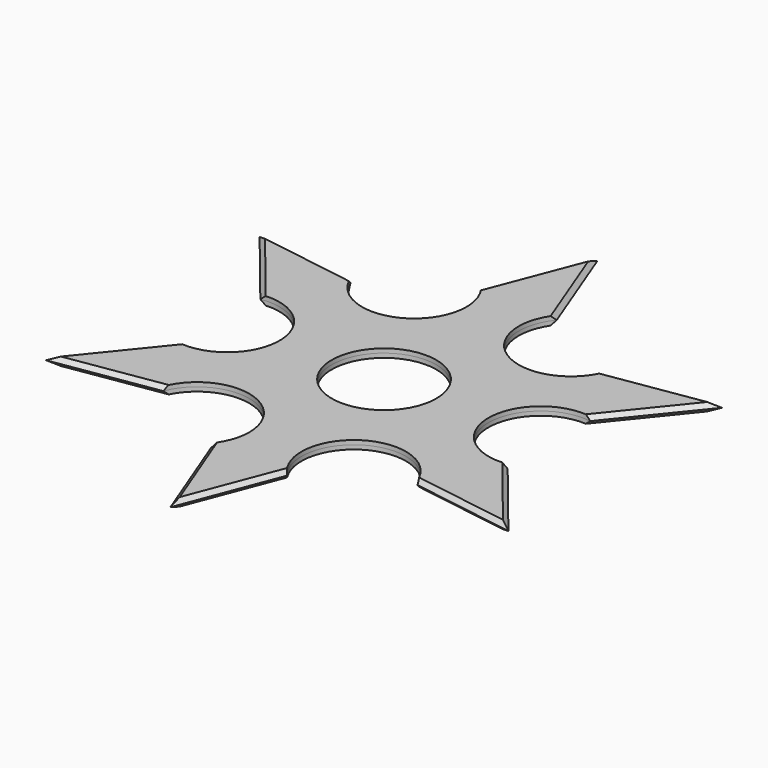
from build123d import *

# Parameters (mm, degrees)
F0_R         = 12.5
F1_DEPTH     = 1
F2_T1_DEPTH  = 53.573606434
F2_T3_DEPTH  = 53.573606434
F2_T5_DEPTH  = 53.5736064345
F2_T7_DEPTH  = 53.5736064338
F2_T9_DEPTH  = 53.573606434
F2_T11_DEPTH = 59.849360607
F2_T13_DEPTH = 53.5916397473
F2_T15_DEPTH = 53.5736064341
F2_T17_DEPTH = 53.573606434
F2_T19_DEPTH = 53.573606434
F2_T21_DEPTH = 59.8387499617
F3_DEPTH     = 1
F4_T1_DEPTH  = 40.7151914942
F4_T3_DEPTH  = 19.123558468
F4_T5_DEPTH  = 40.7151914942
F4_T7_DEPTH  = 19.1235584677
F4_T9_DEPTH  = 59.8387499623
F4_T11_DEPTH = 59.8387499618
F4_T13_DEPTH = 59.8387499617
F4_T15_DEPTH = 59.8387499618
F4_T17_DEPTH = 40.7151914942
F4_T19_DEPTH = 19.1235584677
F4_T21_DEPTH = 40.7151914943
F4_T23_DEPTH = 19.1235584676
F4_T25_DEPTH = 59.828531224
F4_T27_DEPTH = 59.849360607
F5_T1_DEPTH  = 59.8387499611
F5_T3_DEPTH  = 59.838749962
F6_T1_DEPTH  = 52.3772114997


# Not quite as in the source:
# - a fillet or chamfer that OpenCascade refuses, or shapes differently, is made with other operations: its cross-section is extruded or revolved along the edge and cut away or added
# - a feature names something its author has since deleted; it is built from what else it names


with BuildPart() as f1:
    # F0 (on Top) → F1 (new body)
    with BuildSketch(Plane.XY):
        with BuildLine():
            ThreePointArc((12.1993091148, -43.1220058508), (12.5252728209, -21.6360831063), (31.2465952446, -32.1842211044))
            Line((31.2465952446, -32.1842211044), (37.4352447857, -33.1602540379))
            Line((37.4352447857, -33.1602540379), (64.9519052827, -37.5000000012))
            Line((64.9519052827, -37.5000000012), (47.4352447858, -15.8397459622))
            Line((47.4352447858, -15.8397459622), (47.4101819713, -15.8831560303))
            ThreePointArc((47.4101819713, -15.8831560303), (47.4189900332, -15.8568402989), (47.4277834882, -15.830519683))
            Line((47.4277834882, -15.830519683), (43.4956507006, -10.968234711))
            ThreePointArc((43.4956507006, -10.968234711), (25, -3e-10), (43.4956507, 10.9682347114))
            Line((43.4956507, 10.9682347114), (47.4277834882, 15.8305196828))
            ThreePointArc((47.4277834882, 15.8305196828), (47.4189900332, 15.8568402987), (47.4101819713, 15.8831560301))
            Line((47.4101819713, 15.8831560301), (47.4352447858, 15.8397459621))
            Line((47.4352447858, 15.8397459621), (64.9519052853, 37.4999999987))
            Line((64.9519052853, 37.4999999987), (37.4352447862, 33.1602540379))
            Line((37.4352447862, 33.1602540379), (37.4603076002, 33.1168439697))
            ThreePointArc((37.4603076002, 33.1168439697), (37.4419215393, 33.1376298408), (37.4235239447, 33.1584055041))
            Line((37.4235239447, 33.1584055041), (31.2465952455, 32.1842211051))
            ThreePointArc((31.2465952455, 32.1842211051), (12.500000001, 21.6506350947), (12.2490554557, 43.152455816))
            Line((12.2490554557, 43.152455816), (10.0042595438, 48.988925187))
            ThreePointArc((10.0042595437, 48.988925187), (9.9770684942, 48.9944701396), (9.9498743714, 49))
            Line((9.9498743714, 49), (10.0000000003, 49))
            Line((10.0000000003, 49), (3e-10, 75))
            Line((3e-10, 75), (-9.9999999997, 49))
            Line((-9.9999999997, 49), (-9.9498743707, 49))
            ThreePointArc((-9.9498743707, 49), (-9.9770684936, 48.9944701396), (-10.0042595431, 48.988925187))
            Line((-10.0042595431, 48.988925187), (-12.2490554551, 43.1524558158))
            ThreePointArc((-12.2490554551, 43.1524558158), (-12.4999999997, 21.6506350948), (-31.2465952441, 32.1842211045))
            Line((-31.2465952441, 32.1842211045), (-37.4352447851, 33.1602540377))
            Line((-37.4352447851, 33.1602540377), (-64.951905283, 37.5000000002))
            Line((-64.951905283, 37.5000000002), (-47.4352447851, 15.839745962))
            Line((-47.4352447851, 15.839745962), (-47.4101819706, 15.8831560301))
            ThreePointArc((-47.4101819706, 15.8831560301), (-47.4189900325, 15.8568402987), (-47.4277834875, 15.8305196828))
            Line((-47.4277834875, 15.8305196828), (-43.4956506999, 10.9682347111))
            ThreePointArc((-43.4956506999, 10.9682347111), (-24.9999999998, 0), (-43.4956506997, -10.9682347113))
            Line((-43.4956506997, -10.9682347113), (-47.4277834875, -15.830519683))
            ThreePointArc((-47.4277834875, -15.830519683), (-47.4189900326, -15.8568402989), (-47.4101819706, -15.8831560303))
            Line((-47.4101819706, -15.8831560303), (-47.4352447851, -15.8397459622))
            Line((-47.4352447851, -15.8397459622), (-64.9519052836, -37.5))
            Line((-64.9519052836, -37.5), (-37.4352447851, -33.1602540379))
            Line((-37.4352447851, -33.1602540379), (-37.4603075996, -33.1168439699))
            ThreePointArc((-37.4603075996, -33.1168439699), (-37.4419215386, -33.1376298409), (-37.4235239441, -33.1584055043))
            Line((-37.4235239441, -33.1584055043), (-31.2465952444, -32.1842211048))
            ThreePointArc((-31.2465952444, -32.1842211048), (-12.4748304406, -21.6652058125), (-12.2988061822, -43.1825906916))
            Line((-12.2988061822, -43.1825906916), (-10.058717508, -48.977772531))
            ThreePointArc((-10.058717508, -48.977772531), (-10.0043021126, -48.9889164938), (-9.9498743711, -49))
            Line((-9.9498743711, -49), (-10.0501256289, -49))
            Line((-10.0501256289, -49), (0, -75))
            Line((0, -75), (9.9498743711, -49))
            Line((9.9498743711, -49), (12.1993091148, -43.1220058508))
        make_face()
        Circle(F0_R, mode=Mode.SUBTRACT)
    extrude(amount=F1_DEPTH)

    # F2: chamfer of 5 on 11 edges, made by hand

    # F2_s2 → F2_t1 (cut)
    with BuildSketch(Plane(origin=(-10.5129640229, 27.3337064595, 0), x_dir=(0, 0, 1), z_dir=(-0.3589790793, 0.9333456062, 0))):
        Polygon((1, 21.9234309485), (-4, 26.9234309485), (1, 26.9234309485), align=None)
    extrude(amount=F2_T1_DEPTH, mode=Mode.SUBTRACT)

    # F2_s4 → F2_t3 (cut)
    with BuildSketch(Plane(origin=(29.7447679359, 77.3363966333, 0), x_dir=(0, 0, 1), z_dir=(-0.3589790793, -0.9333456062, 0))):
        Polygon((1, 21.9234309479), (-4, 26.9234309479), (1, 26.9234309479), align=None)
    extrude(amount=F2_T3_DEPTH, mode=Mode.SUBTRACT)

    # F2_s6 → F2_t5 (cut)
    with BuildSketch(Plane(origin=(81.84766809, 12.9084736504, 0), x_dir=(0, 0, 1), z_dir=(-0.9877905451, -0.1557878009, 0))):
        Polygon((1, 21.9234309501), (-4, 26.9234309501), (1, 26.9234309501), align=None)
    extrude(amount=F2_T5_DEPTH, mode=Mode.SUBTRACT)

    # F2_s8 → F2_t7 (cut)
    with BuildSketch(Plane(origin=(18.4152021646, 22.771347143, 0), x_dir=(0, 0, 1), z_dir=(0.6288114659, 0.7775578052, 0))):
        Polygon((1, 21.9234309459), (-4, 26.9234309459), (1, 26.9234309459), align=None)
    extrude(amount=F2_T7_DEPTH, mode=Mode.SUBTRACT)

    # F2_s10 → F2_t9 (cut)
    with BuildSketch(Plane(origin=(52.1029001483, -64.427922981, 0), x_dir=(0, 0, 1), z_dir=(-0.6288114658, 0.7775578053, 0))):
        Polygon((1, 21.9234309512), (-4, 26.9234309512), (1, 26.9234309512), align=None)
    extrude(amount=F2_T9_DEPTH, mode=Mode.SUBTRACT)

    # F2_s12 → F2_t11 (cut)
    with BuildSketch(Plane(origin=(-8.2401320813, -21.5322752955, 0), x_dir=(0, 0, 1), z_dir=(-0.3574100383, -0.9339475705, 0))):
        Polygon((1, -21.8057528732), (-4, -26.8057528732), (1, -26.8057528732), align=None)
    extrude(amount=F2_T11_DEPTH, mode=Mode.SUBTRACT)

    # F2_s14 → F2_t13 (cut)
    with BuildSketch(Plane(origin=(10.5359959788, -27.256962307, 0), x_dir=(0, 0, 1), z_dir=(0.3605450827, -0.9327417881, 0))):
        Polygon((1, 22.0408812024), (-4, 27.0408812024), (1, 27.0408812024), align=None)
    extrude(amount=F2_T13_DEPTH, mode=Mode.SUBTRACT)

    # F2_s16 → F2_t15 (cut)
    with BuildSketch(Plane(origin=(-81.8476680892, -12.9084736542, 0), x_dir=(0, 0, 1), z_dir=(0.9877905451, 0.155787801, 0))):
        Polygon((1, 21.9234309484), (-4, 26.9234309484), (1, 26.9234309484), align=None)
    extrude(amount=F2_T15_DEPTH, mode=Mode.SUBTRACT)

    # F2_s18 → F2_t17 (cut)
    with BuildSketch(Plane(origin=(-18.4152021622, -22.7713471426, 0), x_dir=(0, 0, 1), z_dir=(-0.6288114658, -0.7775578052, 0))):
        Polygon((1, 21.9234309477), (-4, 26.9234309477), (1, 26.9234309477), align=None)
    extrude(amount=F2_T17_DEPTH, mode=Mode.SUBTRACT)

    # F2_s20 → F2_t19 (cut)
    with BuildSketch(Plane(origin=(-52.1029001516, 64.4279229792, 0), x_dir=(0, 0, 1), z_dir=(0.6288114658, -0.7775578052, 0))):
        Polygon((1, 21.9234309489), (-4, 26.9234309489), (1, 26.9234309489), align=None)
    extrude(amount=F2_T19_DEPTH, mode=Mode.SUBTRACT)

    # F2_s22 → F2_t21 (cut)
    with BuildSketch(Plane(origin=(-81.8476680889, 12.9084736558, 0), x_dir=(0, 0, 1), z_dir=(0.9877905451, -0.155787801, 0))):
        Polygon((1, -21.9234309474), (-4, -26.9234309474), (1, -26.9234309474), align=None)
    extrude(amount=F2_T21_DEPTH, mode=Mode.SUBTRACT)

    # F6: chamfer of 5 on 1 edges, made by hand

    # F6_s2 → F6_t1 (cut)
    with BuildSketch(Plane(origin=(74.477230945, -11.7460569893, 0), x_dir=(0, 0, 1), z_dir=(-0.9877905451, 0.155787801, 0))):
        Polygon((1, -21.9234309461), (-4, -26.9234309461), (1, -26.9234309461), align=None)
    extrude(amount=F6_T1_DEPTH, mode=Mode.SUBTRACT)


with BuildPart() as f3:
    # F0 (on Top) → F3 (new body)
    with BuildSketch(Plane.XY):
        with BuildLine():
            ThreePointArc((12.1993091148, -43.1220058508), (12.5252728209, -21.6360831063), (31.2465952446, -32.1842211044))
            Line((31.2465952446, -32.1842211044), (37.4352447857, -33.1602540379))
            Line((37.4352447857, -33.1602540379), (64.9519052827, -37.5000000012))
            Line((64.9519052827, -37.5000000012), (47.4352447858, -15.8397459622))
            Line((47.4352447858, -15.8397459622), (47.4101819713, -15.8831560303))
            ThreePointArc((47.4101819713, -15.8831560303), (47.4189900332, -15.8568402989), (47.4277834882, -15.830519683))
            Line((47.4277834882, -15.830519683), (43.4956507006, -10.968234711))
            ThreePointArc((43.4956507006, -10.968234711), (25, -3e-10), (43.4956507, 10.9682347114))
            Line((43.4956507, 10.9682347114), (47.4277834882, 15.8305196828))
            ThreePointArc((47.4277834882, 15.8305196828), (47.4189900332, 15.8568402987), (47.4101819713, 15.8831560301))
            Line((47.4101819713, 15.8831560301), (47.4352447858, 15.8397459621))
            Line((47.4352447858, 15.8397459621), (64.9519052853, 37.4999999987))
            Line((64.9519052853, 37.4999999987), (37.4352447862, 33.1602540379))
            Line((37.4352447862, 33.1602540379), (37.4603076002, 33.1168439697))
            ThreePointArc((37.4603076002, 33.1168439697), (37.4419215393, 33.1376298408), (37.4235239447, 33.1584055041))
            Line((37.4235239447, 33.1584055041), (31.2465952455, 32.1842211051))
            ThreePointArc((31.2465952455, 32.1842211051), (12.500000001, 21.6506350947), (12.2490554557, 43.152455816))
            Line((12.2490554557, 43.152455816), (10.0042595438, 48.988925187))
            ThreePointArc((10.0042595437, 48.988925187), (9.9770684942, 48.9944701396), (9.9498743714, 49))
            Line((9.9498743714, 49), (10.0000000003, 49))
            Line((10.0000000003, 49), (3e-10, 75))
            Line((3e-10, 75), (-9.9999999997, 49))
            Line((-9.9999999997, 49), (-9.9498743707, 49))
            ThreePointArc((-9.9498743707, 49), (-9.9770684936, 48.9944701396), (-10.0042595431, 48.988925187))
            Line((-10.0042595431, 48.988925187), (-12.2490554551, 43.1524558158))
            ThreePointArc((-12.2490554551, 43.1524558158), (-12.4999999997, 21.6506350948), (-31.2465952441, 32.1842211045))
            Line((-31.2465952441, 32.1842211045), (-37.4352447851, 33.1602540377))
            Line((-37.4352447851, 33.1602540377), (-64.951905283, 37.5000000002))
            Line((-64.951905283, 37.5000000002), (-47.4352447851, 15.839745962))
            Line((-47.4352447851, 15.839745962), (-47.4101819706, 15.8831560301))
            ThreePointArc((-47.4101819706, 15.8831560301), (-47.4189900325, 15.8568402987), (-47.4277834875, 15.8305196828))
            Line((-47.4277834875, 15.8305196828), (-43.4956506999, 10.9682347111))
            ThreePointArc((-43.4956506999, 10.9682347111), (-24.9999999998, 0), (-43.4956506997, -10.9682347113))
            Line((-43.4956506997, -10.9682347113), (-47.4277834875, -15.830519683))
            ThreePointArc((-47.4277834875, -15.830519683), (-47.4189900326, -15.8568402989), (-47.4101819706, -15.8831560303))
            Line((-47.4101819706, -15.8831560303), (-47.4352447851, -15.8397459622))
            Line((-47.4352447851, -15.8397459622), (-64.9519052836, -37.5))
            Line((-64.9519052836, -37.5), (-37.4352447851, -33.1602540379))
            Line((-37.4352447851, -33.1602540379), (-37.4603075996, -33.1168439699))
            ThreePointArc((-37.4603075996, -33.1168439699), (-37.4419215386, -33.1376298409), (-37.4235239441, -33.1584055043))
            Line((-37.4235239441, -33.1584055043), (-31.2465952444, -32.1842211048))
            ThreePointArc((-31.2465952444, -32.1842211048), (-12.4748304406, -21.6652058125), (-12.2988061822, -43.1825906916))
            Line((-12.2988061822, -43.1825906916), (-10.058717508, -48.977772531))
            ThreePointArc((-10.058717508, -48.977772531), (-10.0043021126, -48.9889164938), (-9.9498743711, -49))
            Line((-9.9498743711, -49), (-10.0501256289, -49))
            Line((-10.0501256289, -49), (0, -75))
            Line((0, -75), (9.9498743711, -49))
            Line((9.9498743711, -49), (12.1993091148, -43.1220058508))
        make_face()
        Circle(F0_R, mode=Mode.SUBTRACT)
        with BuildLine():
            Line((47.4101819713, -15.8831560303), (47.4352447858, -15.8397459622))
            Line((47.4352447858, -15.8397459622), (47.4277834882, -15.830519683))
            ThreePointArc((47.4277834882, -15.830519683), (47.4189900332, -15.8568402989), (47.4101819713, -15.8831560303))
        make_face()
        with BuildLine():
            Line((-10.058717508, -48.977772531), (-10.0501256289, -49))
            Line((-10.0501256289, -49), (-9.9498743711, -49))
            ThreePointArc((-9.9498743711, -49), (-10.0043021126, -48.9889164938), (-10.058717508, -48.977772531))
        make_face()
        with BuildLine():
            ThreePointArc((47.4101819713, 15.8831560301), (47.4189900332, 15.8568402987), (47.4277834882, 15.8305196828))
            Line((47.4277834882, 15.8305196828), (47.4352447858, 15.8397459621))
            Line((47.4352447858, 15.8397459621), (47.4101819713, 15.8831560301))
        make_face()
        with BuildLine():
            Line((-37.4352447851, -33.1602540379), (-37.4235239441, -33.1584055043))
            ThreePointArc((-37.4235239441, -33.1584055043), (-37.4419215386, -33.1376298409), (-37.4603075996, -33.1168439699))
            Line((-37.4603075996, -33.1168439699), (-37.4352447851, -33.1602540379))
        make_face()
        with BuildLine():
            Line((37.4603076002, 33.1168439697), (37.4352447862, 33.1602540379))
            Line((37.4352447862, 33.1602540379), (37.4235239447, 33.1584055041))
            ThreePointArc((37.4235239447, 33.1584055041), (37.4419215393, 33.1376298408), (37.4603076002, 33.1168439697))
        make_face()
        with BuildLine():
            Line((-47.4277834875, -15.830519683), (-47.4352447851, -15.8397459622))
            Line((-47.4352447851, -15.8397459622), (-47.4101819706, -15.8831560303))
            ThreePointArc((-47.4101819706, -15.8831560303), (-47.4189900326, -15.8568402989), (-47.4277834875, -15.830519683))
        make_face()
        with BuildLine():
            ThreePointArc((9.9498743714, 49), (9.9770684942, 48.9944701396), (10.0042595437, 48.988925187))
            Line((10.0042595438, 48.988925187), (10.0000000003, 49))
            Line((10.0000000003, 49), (9.9498743714, 49))
        make_face()
        with BuildLine():
            Line((-47.4352447851, 15.839745962), (-47.4277834875, 15.8305196828))
            ThreePointArc((-47.4277834875, 15.8305196828), (-47.4189900325, 15.8568402987), (-47.4101819706, 15.8831560301))
            Line((-47.4101819706, 15.8831560301), (-47.4352447851, 15.839745962))
        make_face()
        with BuildLine():
            Line((-9.9498743707, 49), (-9.9999999997, 49))
            Line((-9.9999999997, 49), (-10.0042595431, 48.988925187))
            ThreePointArc((-10.0042595431, 48.988925187), (-9.9770684936, 48.9944701396), (-9.9498743707, 49))
        make_face()
    extrude(amount=-F3_DEPTH)

    # F4: chamfer of 5 on 14 edges, made by hand

    # F4_s2 → F4_t1 (cut)
    with BuildSketch(Plane(origin=(29.7447679359, 77.3363966333, 0), x_dir=(0, 0, 1), z_dir=(-0.3589790793, -0.9333456062, 0))):
        Polygon((4, 26.9234309479), (-1, 21.9234309479), (-1, 26.9234309479), align=None)
    extrude(amount=F4_T1_DEPTH, mode=Mode.SUBTRACT)

    # F4_s4 → F4_t3 (cut)
    with BuildSketch(Plane(origin=(15.1288659793, 39.3350515467, 0), x_dir=(0, 0, 1), z_dir=(-0.3589790793, -0.9333456062, 0))):
        Polygon((4, 26.9234309477), (-1, 21.9234309477), (-1, 26.9234309477), align=None)
    extrude(amount=F4_T3_DEPTH, mode=Mode.SUBTRACT)

    # F4_s6 → F4_t5 (cut)
    with BuildSketch(Plane(origin=(-15.1288659793, 39.3350515463, 0), x_dir=(0, 0, 1), z_dir=(-0.3589790793, 0.9333456062, 0))):
        Polygon((4, 26.9234309485), (-1, 21.9234309485), (-1, 26.9234309485), align=None)
    extrude(amount=F4_T5_DEPTH, mode=Mode.SUBTRACT)

    # F4_s8 → F4_t7 (cut)
    with BuildSketch(Plane(origin=(-8.2639085674, 21.4861622756, 0), x_dir=(0, 0, 1), z_dir=(-0.3589790793, 0.9333456062, 0))):
        Polygon((4, 26.9234309483), (-1, 21.9234309483), (-1, 26.9234309483), align=None)
    extrude(amount=F4_T7_DEPTH, mode=Mode.SUBTRACT)

    # F4_s10 → F4_t9 (cut)
    with BuildSketch(Plane(origin=(81.84766809, 12.9084736504, 0), x_dir=(0, 0, 1), z_dir=(-0.9877905451, -0.1557878009, 0))):
        Polygon((4, 26.9234309501), (-1, 21.9234309501), (-1, 26.9234309501), align=None)
    extrude(amount=F4_T9_DEPTH, mode=Mode.SUBTRACT)

    # F4_s12 → F4_t11 (cut)
    with BuildSketch(Plane(origin=(14.4756080788, 17.8998358922, 0), x_dir=(0, 0, 1), z_dir=(0.6288114659, 0.7775578052, 0))):
        Polygon((4, 26.9234309459), (-1, 21.9234309459), (-1, 26.9234309459), align=None)
    extrude(amount=F4_T11_DEPTH, mode=Mode.SUBTRACT)

    # F4_s14 → F4_t13 (cut)
    with BuildSketch(Plane(origin=(-22.7395166441, 3.5863263841, 0), x_dir=(0, 0, 1), z_dir=(-0.9877905451, 0.155787801, 0))):
        Polygon((4, 26.9234309474), (-1, 21.9234309474), (-1, 26.9234309474), align=None)
    extrude(amount=F4_T13_DEPTH, mode=Mode.SUBTRACT)

    # F4_s16 → F4_t15 (cut)
    with BuildSketch(Plane(origin=(-52.1029001516, 64.4279229792, 0), x_dir=(0, 0, 1), z_dir=(0.6288114658, -0.7775578052, 0))):
        Polygon((4, 26.9234309489), (-1, 21.9234309489), (-1, 26.9234309489), align=None)
    extrude(amount=F4_T15_DEPTH, mode=Mode.SUBTRACT)

    # F4_s18 → F4_t17 (cut)
    with BuildSketch(Plane(origin=(-26.5007209087, -32.7695080417, 0), x_dir=(0, 0, 1), z_dir=(-0.6288114658, -0.7775578052, 0))):
        Polygon((4, 26.9234309477), (-1, 21.9234309477), (-1, 26.9234309477), align=None)
    extrude(amount=F4_T17_DEPTH, mode=Mode.SUBTRACT)

    # F4_s20 → F4_t19 (cut)
    with BuildSketch(Plane(origin=(-14.4756080768, -17.8998358917, 0), x_dir=(0, 0, 1), z_dir=(-0.6288114658, -0.7775578052, 0))):
        Polygon((4, 26.9234309476), (-1, 21.9234309476), (-1, 26.9234309476), align=None)
    extrude(amount=F4_T19_DEPTH, mode=Mode.SUBTRACT)

    # F4_s22 → F4_t21 (cut)
    with BuildSketch(Plane(origin=(-81.8476680892, -12.9084736542, 0), x_dir=(0, 0, 1), z_dir=(0.9877905451, 0.155787801, 0))):
        Polygon((4, 26.9234309484), (-1, 21.9234309484), (-1, 26.9234309484), align=None)
    extrude(amount=F4_T21_DEPTH, mode=Mode.SUBTRACT)

    # F4_s24 → F4_t23 (cut)
    with BuildSketch(Plane(origin=(-41.6295868876, -6.5655435043, 0), x_dir=(0, 0, 1), z_dir=(0.9877905451, 0.155787801, 0))):
        Polygon((4, 26.9234309485), (-1, 21.9234309485), (-1, 26.9234309485), align=None)
    extrude(amount=F4_T23_DEPTH, mode=Mode.SUBTRACT)

    # F4_s26 → F4_t25 (cut)
    with BuildSketch(Plane(origin=(8.2873154255, -21.4395529986, 0), x_dir=(0, 0, 1), z_dir=(0.3605450827, -0.9327417881, 0))):
        Polygon((4, 27.0408812024), (-1, 22.0408812024), (-1, 27.0408812024), align=None)
    extrude(amount=F4_T25_DEPTH, mode=Mode.SUBTRACT)

    # F4_s28 → F4_t27 (cut)
    with BuildSketch(Plane(origin=(-29.6308943486, -77.4284402327, 0), x_dir=(0, 0, 1), z_dir=(0.3574100383, 0.9339475705, 0))):
        Polygon((4, 26.8057528732), (-1, 21.8057528732), (-1, 26.8057528732), align=None)
    extrude(amount=F4_T27_DEPTH, mode=Mode.SUBTRACT)

    # F5: chamfer of 5 on 2 edges, made by hand

    # F5_s2 → F5_t1 (cut)
    with BuildSketch(Plane(origin=(22.7395166453, -3.5863263851, 0), x_dir=(0, 0, 1), z_dir=(0.9877905451, -0.155787801, 0))):
        Polygon((-1, 21.9234309461), (4, 26.9234309461), (-1, 26.9234309461), align=None)
    extrude(amount=F5_T1_DEPTH, mode=Mode.SUBTRACT)

    # F5_s4 → F5_t3 (cut)
    with BuildSketch(Plane(origin=(52.1029001483, -64.427922981, 0), x_dir=(0, 0, 1), z_dir=(-0.6288114658, 0.7775578053, 0))):
        Polygon((-1, 21.9234309512), (4, 26.9234309512), (-1, 26.9234309512), align=None)
    extrude(amount=F5_T3_DEPTH, mode=Mode.SUBTRACT)


solid = Compound([f1.part, f3.part])
